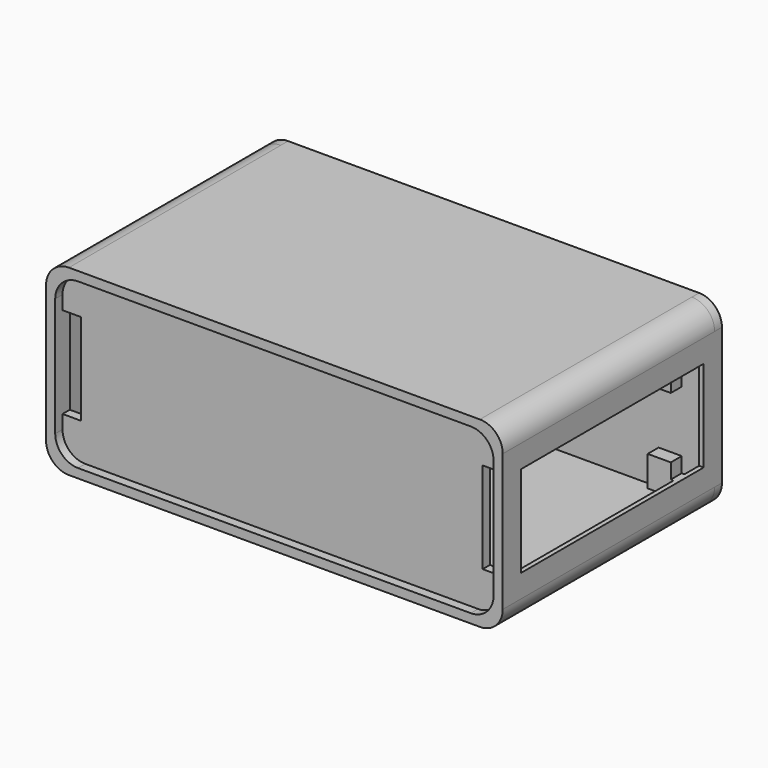
from build123d import *

# Parameters (mm, degrees)
F0_W         = 500
F0_H         = 200
F1_DEPTH     = 150
F2_R         = 25
F4_DEPTH     = 10
F6_DEPTH     = 280
F7_W         = 20
F7_H         = 100
F8_DEPTH     = 10
F9_W         = 25
F9_H         = 10
F9_W_2       = 450
F10_DEPTH    = 200
F11_T1_DEPTH = 134.999500001
F12_W        = 250
F12_H        = 100
F13_DEPTH    = 5
F14_W        = 10
F14_H        = 160
F15_DEPTH    = 10
F16_W        = 15
F16_H        = 16.75
F16_H_2      = 16.55
F17_DEPTH    = 33.3
F18_W        = 15
F18_H        = 16.55
F19_DEPTH    = 8


# Not quite as in the source:
# - a fillet or chamfer that OpenCascade refuses, or shapes differently, is made with other operations: its cross-section is extruded or revolved along the edge and cut away or added
# - a feature names something its author has since deleted; it is built from what else it names


with BuildPart() as f1:
    # F0 (on Front) → F1 (new body, symmetric)
    with BuildSketch(Plane.XZ):
        Rectangle(F0_W, F0_H)
    extrude(amount=F1_DEPTH, both=True)

    # F2
    f2_edges = [f1.edges().sort_by_distance(p)[0] for p in [
        (-250, 0, 100),
        (250, 0, 100),
        (250, 0, -100),
        (-250, 0, -100),
    ]]
    fillet(f2_edges, radius=F2_R)

    # F3 (on face) → F4 (cut)
    with BuildSketch(Plane.XZ.offset(150)):
        with BuildLine():
            ThreePointArc((240, 65), (232.6776695297, 82.6776695297), (215, 90))
            Line((215, 90), (-215, 90))
            ThreePointArc((-215, 90), (-232.6776695297, 82.6776695297), (-240, 65))
            Line((-240, 65), (-240, -65))
            ThreePointArc((-240, -65), (-232.6776695297, -82.6776695297), (-215, -90))
            Line((-215, -90), (215, -90))
            ThreePointArc((215, -90), (232.6776695297, -82.6776695297), (240, -65))
            Line((240, -65), (240, 65))
        make_face()
    extrude(amount=-F4_DEPTH, mode=Mode.SUBTRACT)

    # F5 (on face) → F6 (cut)
    with BuildSketch(Plane(origin=(0, 150, 0), x_dir=(-1, 0, 0), z_dir=(0, 1, 0))):
        with BuildLine():
            ThreePointArc((245, 70), (237.6776695297, 87.6776695297), (220, 95))
            Line((220, 95), (-220, 95))
            ThreePointArc((-220, 95), (-237.6776695297, 87.6776695297), (-245, 70))
            Line((-245, 70), (-245, -70))
            ThreePointArc((-245, -70), (-237.6776695297, -87.6776695297), (-220, -95))
            Line((-220, -95), (220, -95))
            ThreePointArc((220, -95), (237.6776695297, -87.6776695297), (245, -70))
            Line((245, -70), (245, 70))
        make_face()
    extrude(amount=-F6_DEPTH, mode=Mode.SUBTRACT)

    # F7 (on face) → F8 (cut, through all)
    with BuildSketch(Plane.XZ.offset(140)):
        with Locations((-230, 0)):
            Rectangle(F7_W, F7_H)
        with Locations((230, 0)):
            Rectangle(F7_W, F7_H)
    extrude(amount=-F8_DEPTH, mode=Mode.SUBTRACT)

    # F9 (on face) → F10 (join, through all)
    with BuildSketch(Plane.XY.offset(100)):
        with Locations((-237.5, 145)):
            Rectangle(F9_W, F9_H)
        with Locations((0, 145)):
            Rectangle(F9_W_2, F9_H)
        with Locations((237.5, 145)):
            Rectangle(F9_W, F9_H)
    extrude(amount=-F10_DEPTH)

    # F11: fillet of radius 25 on 4 edges, made by hand

    # F11_s2 → F11_t1 (cut)
    with BuildSketch(Plane.XZ.offset(-212.4997500005)):
        with BuildLine():
            ThreePointArc((-250.0001, 75.0001), (-242.6777695297, 92.6777695297), (-225.0001, 100.0001))
            Line((-225.0001, 100.0001), (-225.0001, 100.5001))
            ThreePointArc((-225.0001, 100.5001), (-237.50005, 100.5), (-250, 100.5))
            Line((-250, 100.5), (-250.5, 100))
            ThreePointArc((-250.5, 100), (-250.5, 87.50005), (-250.5001, 75.0001))
            Line((-250.5001, 75.0001), (-250.0001, 75.0001))
        make_face()
        with BuildLine():
            ThreePointArc((-250.0001, -75.0001), (-242.6777695297, -92.6777695297), (-225.0001, -100.0001))
            Line((-225.0001, -100.0001), (-225.0001, -100.5001))
            ThreePointArc((-225.0001, -100.5001), (-237.50005, -100.5), (-250, -100.5))
            Line((-250, -100.5), (-250.5, -100))
            ThreePointArc((-250.5, -100), (-250.5, -87.50005), (-250.5001, -75.0001))
            Line((-250.5001, -75.0001), (-250.0001, -75.0001))
        make_face()
        with BuildLine():
            ThreePointArc((250.0001, 75.0001), (242.6777695297, 92.6777695297), (225.0001, 100.0001))
            Line((225.0001, 100.0001), (225.0001, 100.5001))
            ThreePointArc((225.0001, 100.5001), (237.50005, 100.5), (250, 100.5))
            Line((250, 100.5), (250.5, 100))
            ThreePointArc((250.5, 100), (250.5, 87.50005), (250.5001, 75.0001))
            Line((250.5001, 75.0001), (250.0001, 75.0001))
        make_face()
        with BuildLine():
            ThreePointArc((250.0001, -75.0001), (242.6777695297, -92.6777695297), (225.0001, -100.0001))
            Line((225.0001, -100.0001), (225.0001, -100.5001))
            ThreePointArc((225.0001, -100.5001), (237.50005, -100.5), (250, -100.5))
            Line((250, -100.5), (250.5, -100))
            ThreePointArc((250.5, -100), (250.5, -87.50005), (250.5001, -75.0001))
            Line((250.5001, -75.0001), (250.0001, -75.0001))
        make_face()
    extrude(amount=F11_T1_DEPTH, mode=Mode.SUBTRACT)

    # F12 (on face) → F13 (cut, through all)
    with BuildSketch(Plane.YZ.offset(250)):
        Rectangle(F12_W, F12_H)
    extrude(amount=-F13_DEPTH, mode=Mode.SUBTRACT)

    # F14 (on face) → F15 (cut, through all)
    with BuildSketch(Plane(origin=(0, 150, 0), x_dir=(-1, 0, 0), z_dir=(0, 1, 0))):
        with Locations((35, 0)):
            Rectangle(F14_W, F14_H)
        with Locations((50, 0)):
            Rectangle(F14_W, F14_H)
        with Locations((65, 0)):
            Rectangle(F14_W, F14_H)
        with Locations((80, 0)):
            Rectangle(F14_W, F14_H)
        with Locations((95, 0)):
            Rectangle(F14_W, F14_H)
        with Locations((110, 0)):
            Rectangle(F14_W, F14_H)
        with Locations((125, 0)):
            Rectangle(F14_W, F14_H)
        with Locations((140, 0)):
            Rectangle(F14_W, F14_H)
        with Locations((155, 0)):
            Rectangle(F14_W, F14_H)
        with Locations((170, 0)):
            Rectangle(F14_W, F14_H)
        with Locations((185, 0)):
            Rectangle(F14_W, F14_H)
        with Locations((200, 0)):
            Rectangle(F14_W, F14_H)
        with Locations((215, 0)):
            Rectangle(F14_W, F14_H)
    extrude(amount=-F15_DEPTH, mode=Mode.SUBTRACT)

    # F16 (on face) → F17 (join)
    with BuildSketch(Plane.YZ.offset(250)):
        with Locations((97.5, 58.375)):
            Rectangle(F16_W, F16_H)
        with Locations((97.5, 41.725)):
            Rectangle(F16_W, F16_H_2)
        with Locations((97.5, -41.725)):
            Rectangle(F16_W, F16_H_2)
        with Locations((97.5, -58.375)):
            Rectangle(F16_W, F16_H)
    extrude(amount=-F17_DEPTH)

    # F18 (on face) → F19 (cut)
    with BuildSketch(Plane.YZ.offset(250)):
        with Locations((97.5, 41.725)):
            Rectangle(F18_W, F18_H)
        with Locations((97.5, -41.725)):
            Rectangle(F18_W, F18_H)
    extrude(amount=-F19_DEPTH, mode=Mode.SUBTRACT)


solid = f1.part
